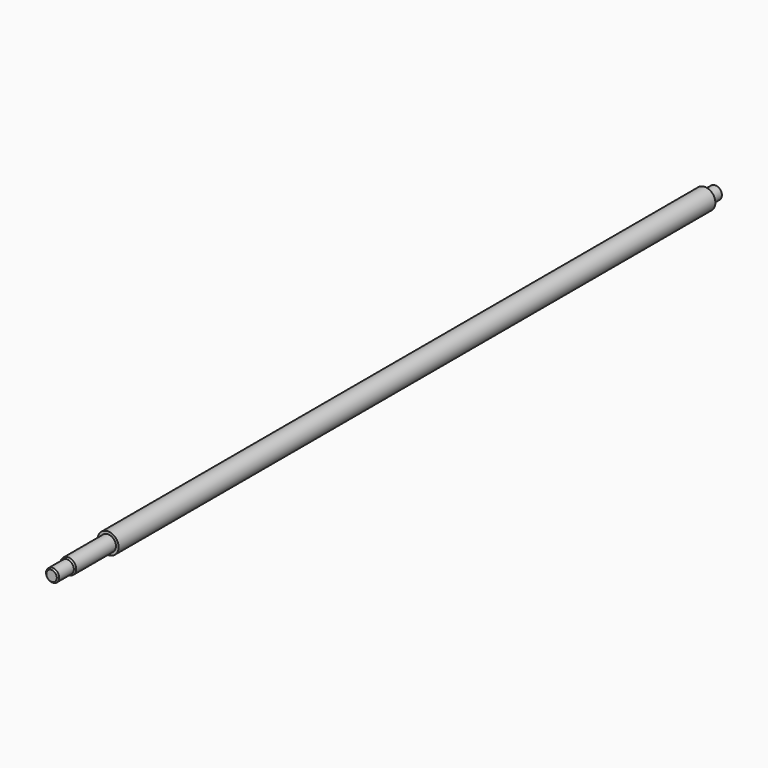
from build123d import *

# Parameters (mm, degrees)
F2_SIZE = 0.99999


# Not quite as in the source:
# - a fillet or chamfer is up to 0.001 mm smaller than in the source, because OpenCascade refuses the exact size


with BuildPart() as f1:
    # F0 (on Right) → F1 (revolve)
    with BuildSketch(Plane.YZ):
        Polygon((0, 5), (0, 0), (635, 0), (635, 5), (624, 5), (624, 8), (54, 8), (54, 6), (15, 6), (15, 5), align=None)
    revolve(axis=Axis((0, 344.1624132916, 0), (0, 1, 0)))

    # F2 (size 1 in the source; OpenCascade refuses exactly that, so slightly less here)
    f2_edges = [f1.edges().sort_by_distance(p)[0] for p in [
        (0, 0, -5),
        (0, 15, -6),
        (0, 635, -5),
    ]]
    chamfer(f2_edges, length=F2_SIZE)


solid = f1.part
